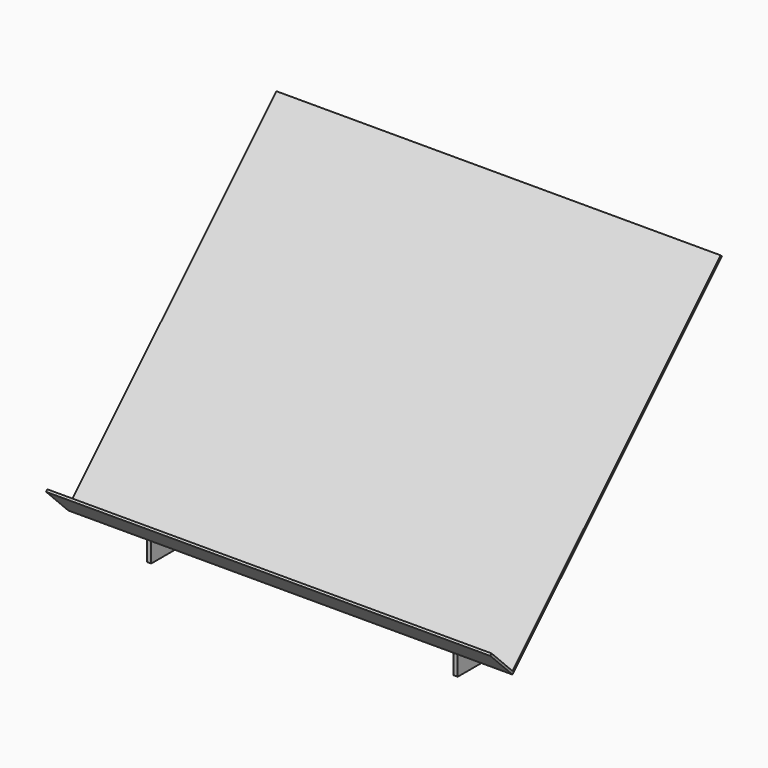
from build123d import *

# Parameters (mm, degrees)
F1_DEPTH = 150
F0_R     = 2.5
F2_DEPTH = 3


with BuildPart() as f1:
    # F0 (on Right) → F1 (new body, symmetric)
    with BuildSketch(Plane.YZ):
        Polygon((-1.0606601718, 1.0606601718), (0, 0), (10, 10), (35, 35), (176.7766952966, 176.7766952966), (175.7160351249, 177.8373554684), (0, 2.1213203436), align=None)
        Polygon((-18.7383297014, 18.7383297014), (-1.0606601718, 1.0606601718), (0, 2.1213203436), (-17.6776695297, 19.7989898732), align=None)
    extrude(amount=F1_DEPTH, both=True)



with BuildPart() as f2:
    # F0 (on Right) → F2 (new body)
    with BuildSketch(Plane.YZ):
        Polygon((35, 35), (10, 10), (10, -20), (35, -20), align=None)
        with Locations((22.5, -10)):
            Circle(F0_R, mode=Mode.SUBTRACT)
        with Locations((22.5, 5)):
            Circle(F0_R, mode=Mode.SUBTRACT)
    extrude(amount=-F2_DEPTH)


with BuildPart() as f2_1:
    # F3: moved
    add(f2.part.moved(Location((105, 0, 0))))


with BuildPart() as f1_1:
    add(f1.part)

    add(f2_1.part)  # F4 merges F2
    # F4: F2 across plane
    add(f2_1.part.mirror(Plane.YZ))


solid = f1_1.part
